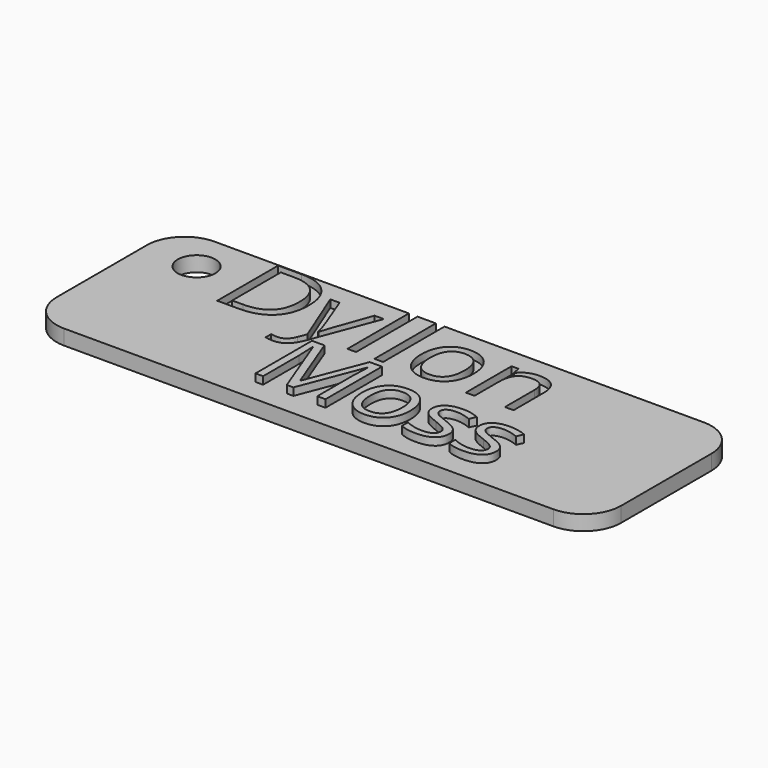
from build123d import *

# Parameters (mm, degrees)
F1_DEPTH     = 2
F3_D         = 5
F4_TEXT_SIZE = 14.1734972648
F5_DEPTH     = 1
F6_TEXT_SIZE = 13.1489075203
F7_DEPTH     = 1


# Not quite as in the source:
# - Text() gives the source's letters only with a copy of the font that has no kerning and outlines rounded to 1/6400 em; it was checked with that copy


with BuildPart() as f1:
    # F0 (on Top) → F1 (new body)
    with BuildSketch(Plane.XY):
        with BuildLine():
            ThreePointArc((37.5, 7.5), (36.0355339059, 11.0355339059), (32.5, 12.5))
            Line((32.5, 12.5), (-32.5, 12.5))
            ThreePointArc((-32.5, 12.5), (-36.0355339059, 11.0355339059), (-37.5, 7.5))
            Line((-37.5, 7.5), (-37.5, -7.5))
            ThreePointArc((-37.5, -7.5), (-36.0355339059, -11.0355339059), (-32.5, -12.5))
            Line((-32.5, -12.5), (32.5, -12.5))
            ThreePointArc((32.5, -12.5), (36.0355339059, -11.0355339059), (37.5, -7.5))
            Line((37.5, -7.5), (37.5, 7.5))
        make_face()
    extrude(amount=F1_DEPTH)

    # F3 (through all)
    with Locations(Plane.XY.offset(2)):
        with Locations((-30.5, 7)):
            Hole(F3_D / 2)

    # F4 (on face) → F5 (cut)
    with BuildSketch(Plane.XY.offset(2)):
        with Locations((-25.3893453628, 2.2950819694)):
            Text('Dyllon', F4_TEXT_SIZE, font='Open Sans', text_align=(TextAlign.LEFT, TextAlign.BOTTOM))
    extrude(amount=-F5_DEPTH, mode=Mode.SUBTRACT)

    # F6 (on face) → F7 (join)
    with BuildSketch(Plane.XY.offset(2)):
        with Locations((-10.7896357989, -9.4672134146)):
            Text('Moss', F6_TEXT_SIZE, font='Open Sans', text_align=(TextAlign.LEFT, TextAlign.BOTTOM))
    extrude(amount=F7_DEPTH)


solid = f1.part
